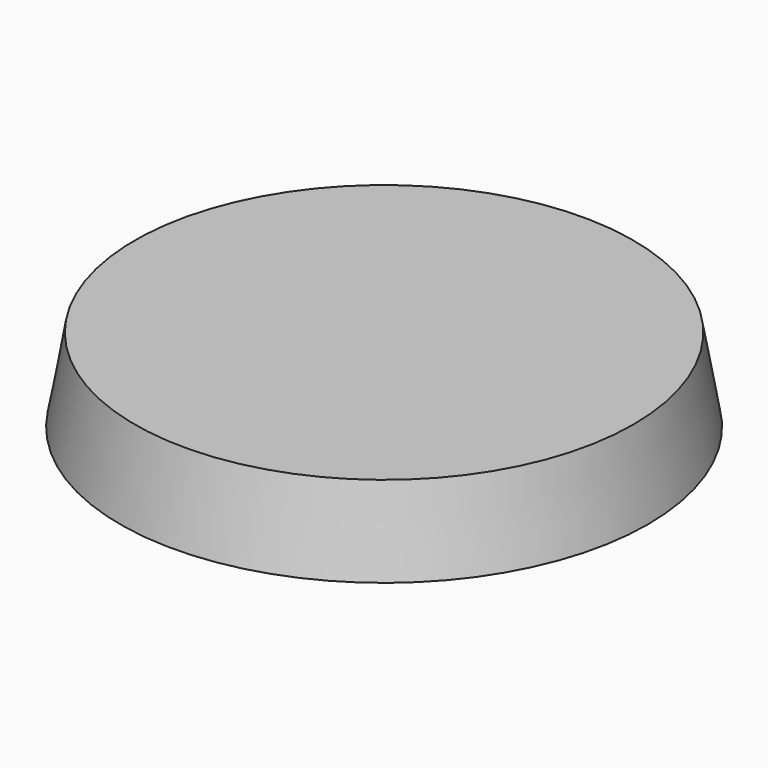
from build123d import *

# Parameters (mm, degrees)
F0_R         = 30
F1_DEPTH     = 10
F1_TAPER     = -10
F2_TEXT_SIZE = 25.8481421648
F3_DEPTH     = 1


# Not quite as in the source:
# - Text() gives the source's letters only with a copy of the font that has no kerning and outlines rounded to 1/6400 em; it was checked with that copy


with BuildPart() as f1:
    # F0 (on Top) → F1 (new body)
    with BuildSketch(Plane.XY):
        Circle(F0_R)
    extrude(amount=-F1_DEPTH, taper=F1_TAPER)

    # F2 (on face) → F3 (cut)
    with BuildSketch(Plane(origin=(0, 0, -10), x_dir=(1, 0, 0), z_dir=(0, 0, -1))):
        with Locations((-27.7818170836, -8.2866894941)):
            Text('Mari', F2_TEXT_SIZE, font='Open Sans', font_style=FontStyle.ITALIC, text_align=(TextAlign.LEFT, TextAlign.BOTTOM))
    extrude(amount=-F3_DEPTH, mode=Mode.SUBTRACT)


solid = f1.part
